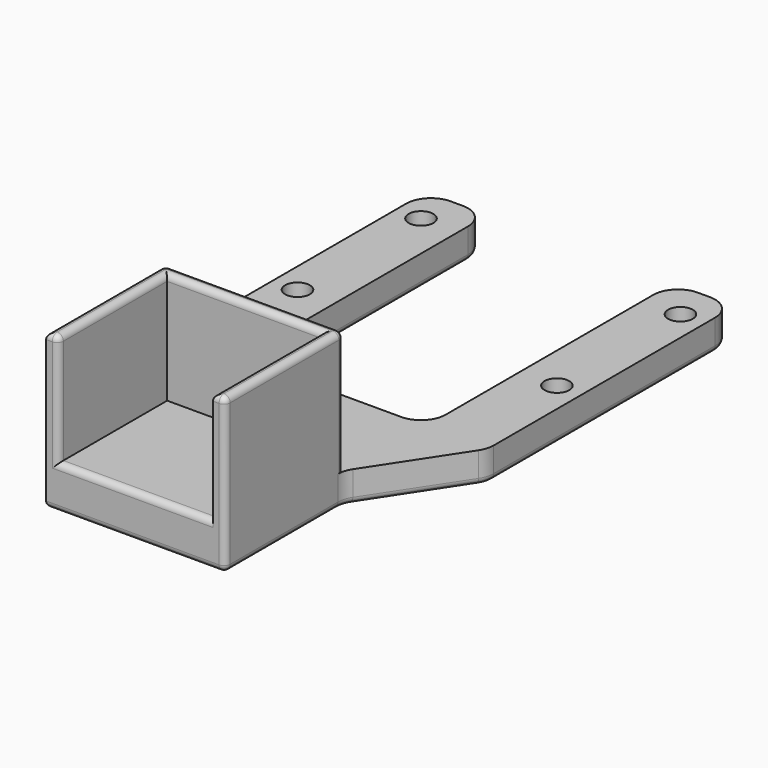
from build123d import *

# Parameters (mm, degrees)
F0_W     = 14.5
F0_H     = 12
F1_DEPTH = 10
F2_W     = 12.5
F2_H     = 11
F3_DEPTH = 9
F4_R     = 1
F5_DEPTH = 2.5
F6_R     = 0.49999


# Not quite as in the source:
# - a fillet or chamfer is up to 0.001 mm smaller than in the source, because OpenCascade refuses the exact size


with BuildPart() as f1:
    # F0 (on Top) → F1 (new body)
    with BuildSketch(Plane.XY):
        with Locations((7.25, 6)):
            Rectangle(F0_W, F0_H)
    extrude(amount=F1_DEPTH)

    # F2 (on face) → F3 (cut)
    with BuildSketch(Plane.XY.offset(10)):
        with Locations((7.25, 5.5)):
            Rectangle(F2_W, F2_H)
    extrude(amount=-F3_DEPTH, mode=Mode.SUBTRACT)

    # F4 (on face) → F5 (join)
    with BuildSketch(Plane(origin=(0, 0, 0), x_dir=(1, 0, 0), z_dir=(0, 0, -1))):
        with BuildLine():
            ThreePointArc((0, -2), (0.5857864376, -0.5857864376), (2, 0))
            Line((2, 0), (0, 0))
            Line((0, 0), (0, -2))
        make_face()
        with BuildLine():
            Line((12.5, 0), (2, 0))
            ThreePointArc((2, 0), (0.5857864376, -0.5857864376), (0, -2))
            Line((0, -2), (0, -11.4023506269))
            ThreePointArc((0, -11.4023506269), (-0.083728667, -11.9749798073), (-0.3279041783, -12.4996635098))
            Line((-0.3279041783, -12.4996635098), (-4.9220958217, -19.5003364902))
            ThreePointArc((-4.9220958217, -19.5003364902), (-5.166271333, -20.0250201927), (-5.25, -20.5976493731))
            Line((-5.25, -20.5976493731), (-5.25, -43))
            ThreePointArc((-5.25, -43), (-4.6642135624, -44.4142135624), (-3.25, -45))
            Line((-3.25, -45), (-2.2500000894, -45))
            ThreePointArc((-2.2500000894, -45), (-0.835786527, -44.4142135624), (-0.2500000894, -43))
            Line((-0.2500000894, -43), (-0.2500000894, -22))
            ThreePointArc((-0.2500000894, -22), (0.3357863482, -20.5857864376), (1.7499999106, -20))
            Line((1.7499999106, -20), (12.7500000894, -20))
            ThreePointArc((12.7500000894, -20), (14.1642136518, -20.5857864376), (14.7500000894, -22))
            Line((14.7500000894, -22), (14.7500000894, -43))
            ThreePointArc((14.7500000894, -43), (15.335786527, -44.4142135624), (16.7500000894, -45))
            Line((16.7500000894, -45), (17.75, -45))
            ThreePointArc((17.75, -45), (19.1642135624, -44.4142135624), (19.75, -43))
            Line((19.75, -43), (19.75, -20.5976493731))
            ThreePointArc((19.75, -20.5976493731), (19.666271333, -20.0250201927), (19.4220958217, -19.5003364902))
            Line((19.4220958217, -19.5003364902), (14.8279041783, -12.4996635098))
            ThreePointArc((14.8279041783, -12.4996635098), (14.583728667, -11.9749798073), (14.5, -11.4023506269))
            Line((14.5, -11.4023506269), (14.5, -2))
            ThreePointArc((14.5, -2), (13.9142135624, -0.5857864376), (12.5, 0))
        make_face()
        with Locations((-3.25, -42)):
            Circle(F4_R, mode=Mode.SUBTRACT)
        with Locations((-3.25, -29.5)):
            Circle(F4_R, mode=Mode.SUBTRACT)
        with Locations((17.75, -42)):
            Circle(F4_R, mode=Mode.SUBTRACT)
        with Locations((17.75, -29.5)):
            Circle(F4_R, mode=Mode.SUBTRACT)
        with BuildLine():
            Line((14.5, 0), (12.5, 0))
            ThreePointArc((12.5, 0), (13.9142135624, -0.5857864376), (14.5, -2))
            Line((14.5, -2), (14.5, 0))
        make_face()
    extrude(amount=F5_DEPTH)

    # F6 (radius 0.5 in the source; OpenCascade refuses exactly that, so slightly less here)
    f6_edges = [f1.edges().sort_by_distance(p)[0] for p in [
        (14.5, 12, 5),
        (0, 12, 5),
        (14.5, 0, 3.75),
        (1, 0, 5.5),
        (14.5, 5.701175, -2.5),
        (0, 5.701175, -2.5),
        (-0.083729, 11.97498, -2.5),
        (-2.625, 16, -2.5),
        (-5.166271, 20.02502, -2.5),
        (-5.25, 31.798825, -2.5),
        (-4.664214, 44.414214, -2.5),
        (-2.75, 45, -2.5),
        (-0.835787, 44.414214, -2.5),
        (-0.25, 32.5, -2.5),
        (0.335786, 20.585786, -2.5),
        (7.25, 20, -2.5),
        (14.164214, 20.585786, -2.5),
        (14.75, 32.5, -2.5),
        (15.335787, 44.414214, -2.5),
        (17.25, 45, -2.5),
        (19.164214, 44.414214, -2.5),
        (19.75, 31.798825, -2.5),
        (19.666271, 20.02502, -2.5),
        (17.125, 16, -2.5),
        (14.583729, 11.97498, -2.5),
        (7.25, 0, -2.5),
        (16.75, 29.5, -2.5),
        (-4.25, 42, -2.5),
        (-4.25, 29.5, -2.5),
        (16.75, 42, -2.5),
        (7.25, 0, 1),
        (0, 6, 10),
        (1, 5.5, 10),
        (7.25, 11, 10),
        (7.25, 12, 10),
        (14.5, 6, 10),
        (14, 0, 10),
        (13.5, 5.5, 10),
        (0.5, 0, 10),
    ]]
    fillet(f6_edges, radius=F6_R)


solid = f1.part
